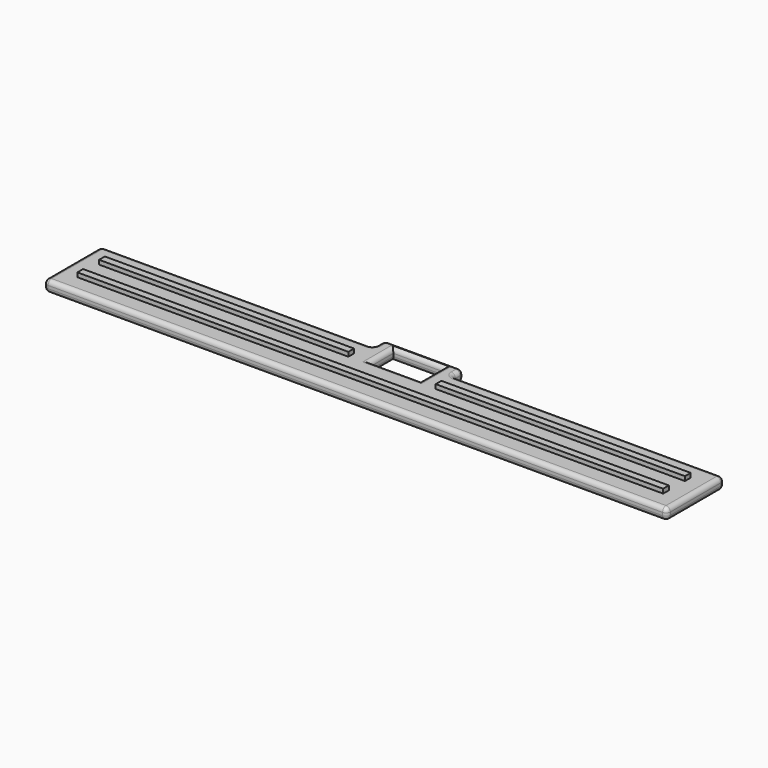
from build123d import *

# Parameters (mm, degrees)
F0_W          = 7
F0_H          = 4
F1_DEPTH      = 1.6
F2_T3_DEPTH   = 1.6
F2_T6_DEPTH   = 1.6
F2_S9_W       = 0.6
F2_S9_H       = 0.6
F2_T10_DEPTH  = 0.6
F2_S14_W      = 0.6
F2_S14_H      = 0.6
F2_T15_DEPTH  = 0.6
F2_S19_W      = 0.6
F2_S19_H      = 0.6
F2_T20_DEPTH  = 0.6
F2_S24_W      = 0.6
F2_S24_H      = 0.6
F2_T25_DEPTH  = 0.6
F2_T30_DEPTH  = 10.9
F2_T33_DEPTH  = 85.8
F2_T36_DEPTH  = 10.9
F2_T39_DEPTH  = 14
F2_T42_DEPTH  = 4
F2_T45_DEPTH  = 7
F2_T48_DEPTH  = 4
F2_T51_DEPTH  = 7
F2_T54_DEPTH  = 10.9
F2_T57_DEPTH  = 85.8
F2_T60_DEPTH  = 10.9
F2_T63_DEPTH  = 14
F2_T66_DEPTH  = 4
F2_T69_DEPTH  = 7
F2_T72_DEPTH  = 4
F2_T75_DEPTH  = 7
F2_T78_DEPTH  = 0.4
F2_T81_DEPTH  = 4.6
F2_T84_DEPTH  = 4.6
F2_T87_DEPTH  = 4.6
F2_T90_DEPTH  = 4.6
F2_T93_DEPTH  = 0.4
F2_T97_DEPTH  = 5.5
F2_T101_DEPTH = 8.5
F2_T107_DEPTH = 5.5
F2_T111_DEPTH = 8.5
F2_T117_DEPTH = 8.5
F2_T121_DEPTH = 5.5
F2_T127_DEPTH = 5.5
F2_T131_DEPTH = 8.5
F2_T137_DEPTH = 5.5
F2_T141_DEPTH = 8.5
F2_T147_DEPTH = 5.5
F2_T151_DEPTH = 8.5
F2_T157_DEPTH = 8.5
F2_T161_DEPTH = 5.5
F2_T167_DEPTH = 5.5
F2_T171_DEPTH = 8.5
F2_S176_W     = 0.6
F2_S176_H     = 0.6
F2_T177_DEPTH = 0.6
F2_S181_W     = 0.6
F2_S181_H     = 0.6
F2_T182_DEPTH = 0.6
F2_S186_W     = 0.6
F2_S186_H     = 0.6
F2_T187_DEPTH = 0.6
F2_S191_W     = 0.6
F2_S191_H     = 0.6
F2_T192_DEPTH = 0.6
F2_S196_W     = 0.6
F2_S196_H     = 0.6
F2_T197_DEPTH = 0.6
F2_S201_W     = 0.6
F2_S201_H     = 0.6
F2_T202_DEPTH = 0.6
F2_S206_W     = 0.6
F2_S206_H     = 0.6
F2_T207_DEPTH = 0.6
F2_S211_W     = 0.6
F2_S211_H     = 0.6
F2_T212_DEPTH = 0.6
F2_T217_DEPTH = 36.8
F2_T220_DEPTH = 0.8
F2_T223_DEPTH = 0.8
F2_T226_DEPTH = 36.8
F2_T229_DEPTH = 36.8
F2_T232_DEPTH = 0.8
F2_T235_DEPTH = 0.8
F2_T238_DEPTH = 36.8
F2_T241_ANGLE = 90
F2_T244_ANGLE = 90
F2_T247_ANGLE = 90
F2_T250_ANGLE = 90
F3_W          = 34.8
F3_H          = 1
F3_W_2        = 81.8
F4_DEPTH      = 2.2


# Not quite as in the source:
# - a fillet or chamfer that OpenCascade refuses, or shapes differently, is made with other operations: its cross-section is extruded or revolved along the edge and cut away or added


with BuildPart() as f1:
    # F0 (on Top) → F1 (new body)
    with BuildSketch(Plane.XY):
        Polygon((-43.5, 10), (-43.5, 0), (43.5, 0), (43.5, 10), (5.5, 10), (5.5, 12), (-5.5, 12), (-5.5, 10), align=None)
        with Locations((0, 9)):
            Rectangle(F0_W, F0_H, mode=Mode.SUBTRACT)
    extrude(amount=F1_DEPTH)

    # F2: fillet of radius 0.6 on 32 edges, made by hand


with BuildPart() as f2_tool1:
    # F2_s2 → F2_t3 (new body)
    with BuildSketch(Plane.XY):
        with BuildLine():
            ThreePointArc((6.1, 10), (5.6757359313, 10.1757359313), (5.5, 10.6))
            Line((5.5, 10.6), (5.5, 10))
            Line((5.5, 10), (6.1, 10))
        make_face()
    extrude(amount=F2_T3_DEPTH)


with BuildPart() as f2_tool4:
    # F2_s5 → F2_t6 (new body)
    with BuildSketch(Plane.XY):
        with BuildLine():
            ThreePointArc((-5.5, 10.6), (-5.6757359313, 10.1757359313), (-6.1, 10))
            Line((-6.1, 10), (-5.5, 10))
            Line((-5.5, 10), (-5.5, 10.6))
        make_face()
    extrude(amount=F2_T6_DEPTH)


with BuildPart() as f1_1:
    add(f1.part)

    # F2_t7: union F2_tool1, F2_tool4
    add([f2_tool1.part, f2_tool4.part])


with BuildPart() as f2_tool8:
    # F2_s9 → F2_t10 (new body)
    with BuildSketch(Plane.YZ.offset(-42.9)):
        with Locations((0.3, 1.3)):
            Rectangle(F2_S9_W, F2_S9_H)
    extrude(amount=-F2_T10_DEPTH)

    # F2_s11 → F2_t12 (revolve, cut)
    with BuildSketch(Plane(origin=(-42.9, 0.6, 1), x_dir=(0, 0.7071067812, -0.7071067812), z_dir=(0, 0.7071067812, 0.7071067812))):
        with BuildLine():
            ThreePointArc((0, -0.6), (0.6, 0), (0, 0.6))
            Line((0, 0.6), (0, -0.6))
        make_face()
    revolve(axis=Axis((-42.9, 0.6, 1), (-1, 0, 0)), mode=Mode.SUBTRACT)


with BuildPart() as f2_tool13:
    # F2_s14 → F2_t15 (new body)
    with BuildSketch(Plane.XZ.offset(-0.6)):
        with Locations((43.2, 1.3)):
            Rectangle(F2_S14_W, F2_S14_H)
    extrude(amount=F2_T15_DEPTH)

    # F2_s16 → F2_t17 (revolve, cut)
    with BuildSketch(Plane(origin=(42.9, 0.6, 1), x_dir=(-0.7071067812, 0, -0.7071067812), z_dir=(-0.7071067812, 0, 0.7071067812))):
        with BuildLine():
            ThreePointArc((0, -0.6), (0.6, 0), (0, 0.6))
            Line((0, 0.6), (0, -0.6))
        make_face()
    revolve(axis=Axis((42.9, 0.6, 1), (0, -1, 0)), mode=Mode.SUBTRACT)


with BuildPart() as f2_tool18:
    # F2_s19 → F2_t20 (new body)
    with BuildSketch(Plane.YZ.offset(-42.9)):
        with Locations((0.3, 0.3)):
            Rectangle(F2_S19_W, F2_S19_H)
    extrude(amount=-F2_T20_DEPTH)

    # F2_s21 → F2_t22 (revolve, cut)
    with BuildSketch(Plane(origin=(-42.9, 0.6, 0.6), x_dir=(0, 0.7071067812, 0.7071067812), z_dir=(0, -0.7071067812, 0.7071067812))):
        with BuildLine():
            ThreePointArc((0, -0.6), (0.6, 0), (0, 0.6))
            Line((0, 0.6), (0, -0.6))
        make_face()
    revolve(axis=Axis((-42.9, 0.6, 0.6), (-1, 0, 0)), mode=Mode.SUBTRACT)


with BuildPart() as f2_tool23:
    # F2_s24 → F2_t25 (new body)
    with BuildSketch(Plane.XZ.offset(-0.6)):
        with Locations((43.2, 0.3)):
            Rectangle(F2_S24_W, F2_S24_H)
    extrude(amount=F2_T25_DEPTH)

    # F2_s26 → F2_t27 (revolve, cut)
    with BuildSketch(Plane(origin=(42.9, 0.6, 0.6), x_dir=(-0.7071067812, 0, 0.7071067812), z_dir=(0.7071067812, 0, 0.7071067812))):
        with BuildLine():
            ThreePointArc((0, -0.6), (0.6, 0), (0, 0.6))
            Line((0, 0.6), (0, -0.6))
        make_face()
    revolve(axis=Axis((42.9, 0.6, 0.6), (0, -1, 0)), mode=Mode.SUBTRACT)


with BuildPart() as f2_tool28:
    # F2_s29 → F2_t30 (new body)
    with BuildSketch(Plane.XZ.offset(-11.5)):
        with BuildLine():
            ThreePointArc((-43.5, 1), (-43.3242640687, 1.4242640687), (-42.9, 1.6))
            Line((-42.9, 1.6), (-43.5, 1.6))
            Line((-43.5, 1.6), (-43.5, 1))
        make_face()
    extrude(amount=F2_T30_DEPTH)


with BuildPart() as f2_tool31:
    # F2_s32 → F2_t33 (new body)
    with BuildSketch(Plane.YZ.offset(-42.9)):
        with BuildLine():
            ThreePointArc((0, 1), (0.1757359313, 1.4242640687), (0.6, 1.6))
            Line((0.6, 1.6), (0, 1.6))
            Line((0, 1.6), (0, 1))
        make_face()
    extrude(amount=F2_T33_DEPTH)


with BuildPart() as f2_tool34:
    # F2_s35 → F2_t36 (new body)
    with BuildSketch(Plane.XZ.offset(-0.6)):
        with BuildLine():
            ThreePointArc((42.9, 1.6), (43.3242640687, 1.4242640687), (43.5, 1))
            Line((43.5, 1), (43.5, 1.6))
            Line((43.5, 1.6), (42.9, 1.6))
        make_face()
    extrude(amount=-F2_T36_DEPTH)


with BuildPart() as f2_tool37:
    # F2_s38 → F2_t39 (new body)
    with BuildSketch(Plane.YZ.offset(7)):
        with BuildLine():
            ThreePointArc((11.4, 1.6), (11.8242640687, 1.4242640687), (12, 1))
            Line((12, 1), (12, 1.6))
            Line((12, 1.6), (11.4, 1.6))
        make_face()
    extrude(amount=-F2_T39_DEPTH)


with BuildPart() as f2_tool40:
    # F2_s41 → F2_t42 (new body)
    with BuildSketch(Plane.XZ.offset(-7)):
        with BuildLine():
            ThreePointArc((-4.1, 1.6), (-3.6757359313, 1.4242640687), (-3.5, 1))
            Line((-3.5, 1), (-3.5, 1.6))
            Line((-3.5, 1.6), (-4.1, 1.6))
        make_face()
    extrude(amount=-F2_T42_DEPTH)


with BuildPart() as f2_tool43:
    # F2_s44 → F2_t45 (new body)
    with BuildSketch(Plane.YZ.offset(-3.5)):
        with BuildLine():
            ThreePointArc((11.6, 1.6), (11.1757359313, 1.4242640687), (11, 1))
            Line((11, 1), (11, 1.6))
            Line((11, 1.6), (11.6, 1.6))
        make_face()
    extrude(amount=F2_T45_DEPTH)


with BuildPart() as f2_tool46:
    # F2_s47 → F2_t48 (new body)
    with BuildSketch(Plane.XZ.offset(-11)):
        with BuildLine():
            ThreePointArc((4.1, 1.6), (3.6757359313, 1.4242640687), (3.5, 1))
            Line((3.5, 1), (3.5, 1.6))
            Line((3.5, 1.6), (4.1, 1.6))
        make_face()
    extrude(amount=F2_T48_DEPTH)


with BuildPart() as f2_tool49:
    # F2_s50 → F2_t51 (new body)
    with BuildSketch(Plane.YZ.offset(3.5)):
        with BuildLine():
            ThreePointArc((6.4, 1.6), (6.8242640687, 1.4242640687), (7, 1))
            Line((7, 1), (7, 1.6))
            Line((7, 1.6), (6.4, 1.6))
        make_face()
    extrude(amount=-F2_T51_DEPTH)


with BuildPart() as f2_tool52:
    # F2_s53 → F2_t54 (new body)
    with BuildSketch(Plane.XZ.offset(-11.5)):
        with BuildLine():
            ThreePointArc((-43.5, 0.6), (-43.3242640687, 0.1757359313), (-42.9, 0))
            Line((-42.9, 0), (-43.5, 0))
            Line((-43.5, 0), (-43.5, 0.6))
        make_face()
    extrude(amount=F2_T54_DEPTH)


with BuildPart() as f2_tool55:
    # F2_s56 → F2_t57 (new body)
    with BuildSketch(Plane.YZ.offset(-42.9)):
        with BuildLine():
            ThreePointArc((0, 0.6), (0.1757359313, 0.1757359313), (0.6, 0))
            Line((0.6, 0), (0, 0))
            Line((0, 0), (0, 0.6))
        make_face()
    extrude(amount=F2_T57_DEPTH)


with BuildPart() as f2_tool58:
    # F2_s59 → F2_t60 (new body)
    with BuildSketch(Plane.XZ.offset(-0.6)):
        with BuildLine():
            ThreePointArc((42.9, 0), (43.3242640687, 0.1757359313), (43.5, 0.6))
            Line((43.5, 0.6), (43.5, 0))
            Line((43.5, 0), (42.9, 0))
        make_face()
    extrude(amount=-F2_T60_DEPTH)


with BuildPart() as f2_tool61:
    # F2_s62 → F2_t63 (new body)
    with BuildSketch(Plane.YZ.offset(7)):
        with BuildLine():
            ThreePointArc((11.4, 0), (11.8242640687, 0.1757359313), (12, 0.6))
            Line((12, 0.6), (12, 0))
            Line((12, 0), (11.4, 0))
        make_face()
    extrude(amount=-F2_T63_DEPTH)


with BuildPart() as f2_tool64:
    # F2_s65 → F2_t66 (new body)
    with BuildSketch(Plane.XZ.offset(-7)):
        with BuildLine():
            ThreePointArc((-4.1, 0), (-3.6757359313, 0.1757359313), (-3.5, 0.6))
            Line((-3.5, 0.6), (-3.5, 0))
            Line((-3.5, 0), (-4.1, 0))
        make_face()
    extrude(amount=-F2_T66_DEPTH)


with BuildPart() as f2_tool67:
    # F2_s68 → F2_t69 (new body)
    with BuildSketch(Plane.YZ.offset(-3.5)):
        with BuildLine():
            ThreePointArc((11.6, 0), (11.1757359313, 0.1757359313), (11, 0.6))
            Line((11, 0.6), (11, 0))
            Line((11, 0), (11.6, 0))
        make_face()
    extrude(amount=F2_T69_DEPTH)


with BuildPart() as f2_tool70:
    # F2_s71 → F2_t72 (new body)
    with BuildSketch(Plane.XZ.offset(-11)):
        with BuildLine():
            ThreePointArc((4.1, 0), (3.6757359313, 0.1757359313), (3.5, 0.6))
            Line((3.5, 0.6), (3.5, 0))
            Line((3.5, 0), (4.1, 0))
        make_face()
    extrude(amount=F2_T72_DEPTH)


with BuildPart() as f2_tool73:
    # F2_s74 → F2_t75 (new body)
    with BuildSketch(Plane.YZ.offset(3.5)):
        with BuildLine():
            ThreePointArc((6.4, 0), (6.8242640687, 0.1757359313), (7, 0.6))
            Line((7, 0.6), (7, 0))
            Line((7, 0), (6.4, 0))
        make_face()
    extrude(amount=-F2_T75_DEPTH)


with BuildPart() as f2_tool76:
    # F2_s77 → F2_t78 (new body)
    with BuildSketch(Plane.XY.offset(0.6)):
        with BuildLine():
            ThreePointArc((42.9, 0), (43.3242640687, 0.1757359313), (43.5, 0.6))
            Line((43.5, 0.6), (43.5, 0))
            Line((43.5, 0), (42.9, 0))
        make_face()
    extrude(amount=F2_T78_DEPTH)


with BuildPart() as f2_tool79:
    # F2_s80 → F2_t81 (new body)
    with BuildSketch(Plane.XY.offset(-1.5)):
        with BuildLine():
            ThreePointArc((43.5, 9.4), (43.3242640687, 9.8242640687), (42.9, 10))
            Line((42.9, 10), (43.5, 10))
            Line((43.5, 10), (43.5, 9.4))
        make_face()
    extrude(amount=F2_T81_DEPTH)


with BuildPart() as f2_tool82:
    # F2_s83 → F2_t84 (new body)
    with BuildSketch(Plane.XY.offset(-1.5)):
        with BuildLine():
            ThreePointArc((5.5, 11.4), (5.3242640687, 11.8242640687), (4.9, 12))
            Line((4.9, 12), (5.5, 12))
            Line((5.5, 12), (5.5, 11.4))
        make_face()
    extrude(amount=F2_T84_DEPTH)


with BuildPart() as f2_tool85:
    # F2_s86 → F2_t87 (new body)
    with BuildSketch(Plane.XY.offset(-1.5)):
        with BuildLine():
            ThreePointArc((-4.9, 12), (-5.3242640687, 11.8242640687), (-5.5, 11.4))
            Line((-5.5, 11.4), (-5.5, 12))
            Line((-5.5, 12), (-4.9, 12))
        make_face()
    extrude(amount=F2_T87_DEPTH)


with BuildPart() as f2_tool88:
    # F2_s89 → F2_t90 (new body)
    with BuildSketch(Plane.XY.offset(-1.5)):
        with BuildLine():
            ThreePointArc((-43.5, 9.4), (-43.3242640687, 9.8242640687), (-42.9, 10))
            Line((-42.9, 10), (-43.5, 10))
            Line((-43.5, 10), (-43.5, 9.4))
        make_face()
    extrude(amount=F2_T90_DEPTH)


with BuildPart() as f2_tool91:
    # F2_s92 → F2_t93 (new body)
    with BuildSketch(Plane.XY.offset(0.6)):
        with BuildLine():
            ThreePointArc((-43.5, 0.6), (-43.3242640687, 0.1757359313), (-42.9, 0))
            Line((-42.9, 0), (-43.5, 0))
            Line((-43.5, 0), (-43.5, 0.6))
        make_face()
    extrude(amount=F2_T93_DEPTH)


with BuildPart() as f2_tool95:
    # F2_s96 → F2_t97 (new body)
    with BuildSketch(Plane.XZ.offset(-5.5)):
        with BuildLine():
            ThreePointArc((-4.1, 1.6), (-3.6757359313, 1.4242640687), (-3.5, 1))
            Line((-3.5, 1), (-3.5, 1.6))
            Line((-3.5, 1.6), (-4.1, 1.6))
        make_face()
    extrude(amount=-F2_T97_DEPTH)

    split(bisect_by=Plane.XZ.offset(-7), keep=Keep.TOP)


with BuildPart() as f2_tool99:
    # F2_s100 → F2_t101 (new body)
    with BuildSketch(Plane.YZ.offset(3.5)):
        with BuildLine():
            ThreePointArc((6.4, 1.6), (6.8242640687, 1.4242640687), (7, 1))
            Line((7, 1), (7, 1.6))
            Line((7, 1.6), (6.4, 1.6))
        make_face()
    extrude(amount=-F2_T101_DEPTH)

    split(bisect_by=Plane.YZ.offset(-3.5), keep=Keep.BOTTOM)


with BuildPart() as f2_tool95_1:
    add(f2_tool95.part)

    # F2_t103: intersect F2_tool99
    add(f2_tool99.part, mode=Mode.INTERSECT)


with BuildPart() as f2_tool105:
    # F2_s106 → F2_t107 (new body)
    with BuildSketch(Plane.XZ.offset(-7)):
        with BuildLine():
            ThreePointArc((-4.1, 1.6), (-3.6757359313, 1.4242640687), (-3.5, 1))
            Line((-3.5, 1), (-3.5, 1.6))
            Line((-3.5, 1.6), (-4.1, 1.6))
        make_face()
    extrude(amount=-F2_T107_DEPTH)

    split(bisect_by=Plane.XZ.offset(-11), keep=Keep.BOTTOM)


with BuildPart() as f2_tool109:
    # F2_s110 → F2_t111 (new body)
    with BuildSketch(Plane.YZ.offset(-5)):
        with BuildLine():
            ThreePointArc((11.6, 1.6), (11.1757359313, 1.4242640687), (11, 1))
            Line((11, 1), (11, 1.6))
            Line((11, 1.6), (11.6, 1.6))
        make_face()
    extrude(amount=F2_T111_DEPTH)

    split(bisect_by=Plane.YZ.offset(-3.5), keep=Keep.BOTTOM)


with BuildPart() as f2_tool105_1:
    add(f2_tool105.part)

    # F2_t113: intersect F2_tool109
    add(f2_tool109.part, mode=Mode.INTERSECT)


with BuildPart() as f2_tool115:
    # F2_s116 → F2_t117 (new body)
    with BuildSketch(Plane.YZ.offset(-3.5)):
        with BuildLine():
            ThreePointArc((11.6, 1.6), (11.1757359313, 1.4242640687), (11, 1))
            Line((11, 1), (11, 1.6))
            Line((11, 1.6), (11.6, 1.6))
        make_face()
    extrude(amount=F2_T117_DEPTH)

    split(bisect_by=Plane.YZ.offset(3.5), keep=Keep.TOP)


with BuildPart() as f2_tool119:
    # F2_s120 → F2_t121 (new body)
    with BuildSketch(Plane.XZ.offset(-12.5)):
        with BuildLine():
            ThreePointArc((4.1, 1.6), (3.6757359313, 1.4242640687), (3.5, 1))
            Line((3.5, 1), (3.5, 1.6))
            Line((3.5, 1.6), (4.1, 1.6))
        make_face()
    extrude(amount=F2_T121_DEPTH)

    split(bisect_by=Plane.XZ.offset(-11), keep=Keep.BOTTOM)


with BuildPart() as f2_tool115_1:
    add(f2_tool115.part)

    # F2_t123: intersect F2_tool119
    add(f2_tool119.part, mode=Mode.INTERSECT)


with BuildPart() as f2_tool125:
    # F2_s126 → F2_t127 (new body)
    with BuildSketch(Plane.XZ.offset(-11)):
        with BuildLine():
            ThreePointArc((4.1, 1.6), (3.6757359313, 1.4242640687), (3.5, 1))
            Line((3.5, 1), (3.5, 1.6))
            Line((3.5, 1.6), (4.1, 1.6))
        make_face()
    extrude(amount=F2_T127_DEPTH)

    split(bisect_by=Plane.XZ.offset(-7), keep=Keep.TOP)


with BuildPart() as f2_tool129:
    # F2_s130 → F2_t131 (new body)
    with BuildSketch(Plane.YZ.offset(5)):
        with BuildLine():
            ThreePointArc((6.4, 1.6), (6.8242640687, 1.4242640687), (7, 1))
            Line((7, 1), (7, 1.6))
            Line((7, 1.6), (6.4, 1.6))
        make_face()
    extrude(amount=-F2_T131_DEPTH)

    split(bisect_by=Plane.YZ.offset(3.5), keep=Keep.TOP)


with BuildPart() as f2_tool125_1:
    add(f2_tool125.part)

    # F2_t133: intersect F2_tool129
    add(f2_tool129.part, mode=Mode.INTERSECT)


with BuildPart() as f2_tool135:
    # F2_s136 → F2_t137 (new body)
    with BuildSketch(Plane.XZ.offset(-5.5)):
        with BuildLine():
            ThreePointArc((-4.1, 0), (-3.6757359313, 0.1757359313), (-3.5, 0.6))
            Line((-3.5, 0.6), (-3.5, 0))
            Line((-3.5, 0), (-4.1, 0))
        make_face()
    extrude(amount=-F2_T137_DEPTH)

    split(bisect_by=Plane.XZ.offset(-7), keep=Keep.TOP)


with BuildPart() as f2_tool139:
    # F2_s140 → F2_t141 (new body)
    with BuildSketch(Plane.YZ.offset(3.5)):
        with BuildLine():
            ThreePointArc((6.4, 0), (6.8242640687, 0.1757359313), (7, 0.6))
            Line((7, 0.6), (7, 0))
            Line((7, 0), (6.4, 0))
        make_face()
    extrude(amount=-F2_T141_DEPTH)

    split(bisect_by=Plane.YZ.offset(-3.5), keep=Keep.BOTTOM)


with BuildPart() as f2_tool135_1:
    add(f2_tool135.part)

    # F2_t143: intersect F2_tool139
    add(f2_tool139.part, mode=Mode.INTERSECT)


with BuildPart() as f2_tool145:
    # F2_s146 → F2_t147 (new body)
    with BuildSketch(Plane.XZ.offset(-7)):
        with BuildLine():
            ThreePointArc((-4.1, 0), (-3.6757359313, 0.1757359313), (-3.5, 0.6))
            Line((-3.5, 0.6), (-3.5, 0))
            Line((-3.5, 0), (-4.1, 0))
        make_face()
    extrude(amount=-F2_T147_DEPTH)

    split(bisect_by=Plane.XZ.offset(-11), keep=Keep.BOTTOM)


with BuildPart() as f2_tool149:
    # F2_s150 → F2_t151 (new body)
    with BuildSketch(Plane.YZ.offset(-5)):
        with BuildLine():
            ThreePointArc((11.6, 0), (11.1757359313, 0.1757359313), (11, 0.6))
            Line((11, 0.6), (11, 0))
            Line((11, 0), (11.6, 0))
        make_face()
    extrude(amount=F2_T151_DEPTH)

    split(bisect_by=Plane.YZ.offset(-3.5), keep=Keep.BOTTOM)


with BuildPart() as f2_tool145_1:
    add(f2_tool145.part)

    # F2_t153: intersect F2_tool149
    add(f2_tool149.part, mode=Mode.INTERSECT)


with BuildPart() as f2_tool155:
    # F2_s156 → F2_t157 (new body)
    with BuildSketch(Plane.YZ.offset(-3.5)):
        with BuildLine():
            ThreePointArc((11.6, 0), (11.1757359313, 0.1757359313), (11, 0.6))
            Line((11, 0.6), (11, 0))
            Line((11, 0), (11.6, 0))
        make_face()
    extrude(amount=F2_T157_DEPTH)

    split(bisect_by=Plane.YZ.offset(3.5), keep=Keep.TOP)


with BuildPart() as f2_tool159:
    # F2_s160 → F2_t161 (new body)
    with BuildSketch(Plane.XZ.offset(-12.5)):
        with BuildLine():
            ThreePointArc((4.1, 0), (3.6757359313, 0.1757359313), (3.5, 0.6))
            Line((3.5, 0.6), (3.5, 0))
            Line((3.5, 0), (4.1, 0))
        make_face()
    extrude(amount=F2_T161_DEPTH)

    split(bisect_by=Plane.XZ.offset(-11), keep=Keep.BOTTOM)


with BuildPart() as f2_tool155_1:
    add(f2_tool155.part)

    # F2_t163: intersect F2_tool159
    add(f2_tool159.part, mode=Mode.INTERSECT)


with BuildPart() as f2_tool165:
    # F2_s166 → F2_t167 (new body)
    with BuildSketch(Plane.XZ.offset(-11)):
        with BuildLine():
            ThreePointArc((4.1, 0), (3.6757359313, 0.1757359313), (3.5, 0.6))
            Line((3.5, 0.6), (3.5, 0))
            Line((3.5, 0), (4.1, 0))
        make_face()
    extrude(amount=F2_T167_DEPTH)

    split(bisect_by=Plane.XZ.offset(-7), keep=Keep.TOP)


with BuildPart() as f2_tool169:
    # F2_s170 → F2_t171 (new body)
    with BuildSketch(Plane.YZ.offset(5)):
        with BuildLine():
            ThreePointArc((6.4, 0), (6.8242640687, 0.1757359313), (7, 0.6))
            Line((7, 0.6), (7, 0))
            Line((7, 0), (6.4, 0))
        make_face()
    extrude(amount=-F2_T171_DEPTH)

    split(bisect_by=Plane.YZ.offset(3.5), keep=Keep.TOP)


with BuildPart() as f2_tool165_1:
    add(f2_tool165.part)

    # F2_t173: intersect F2_tool169
    add(f2_tool169.part, mode=Mode.INTERSECT)


with BuildPart() as f1_2:
    add(f1_1.part)

    # F2_t174: cut F2_tool8, F2_tool13, F2_tool18, F2_tool23, F2_tool28, F2_tool31, F2_tool34, F2_tool37, F2_tool40, F2_tool43, F2_tool46, F2_tool49, F2_tool52, F2_tool55, F2_tool58, F2_tool61, F2_tool64, F2_tool67, F2_tool70, F2_tool73, F2_tool76, F2_tool79, F2_tool82, F2_tool85, F2_tool88, F2_tool91, F2_tool95, F2_tool105, F2_tool115, F2_tool125, F2_tool135, F2_tool145, F2_tool155, F2_tool165
    add([f2_tool8.part, f2_tool13.part, f2_tool18.part, f2_tool23.part, f2_tool28.part, f2_tool31.part, f2_tool34.part, f2_tool37.part, f2_tool40.part, f2_tool43.part, f2_tool46.part, f2_tool49.part, f2_tool52.part, f2_tool55.part, f2_tool58.part, f2_tool61.part, f2_tool64.part, f2_tool67.part, f2_tool70.part, f2_tool73.part, f2_tool76.part, f2_tool79.part, f2_tool82.part, f2_tool85.part, f2_tool88.part, f2_tool91.part, f2_tool95_1.part, f2_tool105_1.part, f2_tool115_1.part, f2_tool125_1.part, f2_tool135_1.part, f2_tool145_1.part, f2_tool155_1.part, f2_tool165_1.part], mode=Mode.SUBTRACT)


with BuildPart() as f2_tool175:
    # F2_s176 → F2_t177 (new body)
    with BuildSketch(Plane.XZ.offset(-9.4)):
        with Locations((-43.2, 0.3)):
            Rectangle(F2_S176_W, F2_S176_H)
    extrude(amount=-F2_T177_DEPTH)

    # F2_s178 → F2_t179 (revolve, cut)
    with BuildSketch(Plane(origin=(-42.9, 9.4, 0.6), x_dir=(0.7071067812, 0, 0.7071067812), z_dir=(-0.7071067812, 0, 0.7071067812))):
        with BuildLine():
            ThreePointArc((0, -0.6), (0.6, 0), (0, 0.6))
            Line((0, 0.6), (0, -0.6))
        make_face()
    revolve(axis=Axis((-42.9, 9.4, 0.6), (0, 1, 0)), mode=Mode.SUBTRACT)


with BuildPart() as f2_tool180:
    # F2_s181 → F2_t182 (new body)
    with BuildSketch(Plane.YZ.offset(-4.9)):
        with Locations((11.7, 0.3)):
            Rectangle(F2_S181_W, F2_S181_H)
    extrude(amount=-F2_T182_DEPTH)

    # F2_s183 → F2_t184 (revolve, cut)
    with BuildSketch(Plane(origin=(-4.9, 11.4, 0.6), x_dir=(0, -0.7071067812, 0.7071067812), z_dir=(0, -0.7071067812, -0.7071067812))):
        with BuildLine():
            ThreePointArc((0, -0.6), (0.6, 0), (0, 0.6))
            Line((0, 0.6), (0, -0.6))
        make_face()
    revolve(axis=Axis((-4.9, 11.4, 0.6), (-1, 0, 0)), mode=Mode.SUBTRACT)


with BuildPart() as f2_tool185:
    # F2_s186 → F2_t187 (new body)
    with BuildSketch(Plane.YZ.offset(4.9)):
        with Locations((11.7, 0.3)):
            Rectangle(F2_S186_W, F2_S186_H)
    extrude(amount=F2_T187_DEPTH)

    # F2_s188 → F2_t189 (revolve, cut)
    with BuildSketch(Plane(origin=(4.9, 11.4, 0.6), x_dir=(0, -0.7071067812, 0.7071067812), z_dir=(0, 0.7071067812, 0.7071067812))):
        with BuildLine():
            ThreePointArc((0, -0.6), (0.6, 0), (0, 0.6))
            Line((0, 0.6), (0, -0.6))
        make_face()
    revolve(axis=Axis((4.9, 11.4, 0.6), (1, 0, 0)), mode=Mode.SUBTRACT)


with BuildPart() as f2_tool190:
    # F2_s191 → F2_t192 (new body)
    with BuildSketch(Plane.XZ.offset(-9.4)):
        with Locations((43.2, 0.3)):
            Rectangle(F2_S191_W, F2_S191_H)
    extrude(amount=-F2_T192_DEPTH)

    # F2_s193 → F2_t194 (revolve, cut)
    with BuildSketch(Plane(origin=(42.9, 9.4, 0.6), x_dir=(-0.7071067812, 0, 0.7071067812), z_dir=(-0.7071067812, 0, -0.7071067812))):
        with BuildLine():
            ThreePointArc((0, -0.6), (0.6, 0), (0, 0.6))
            Line((0, 0.6), (0, -0.6))
        make_face()
    revolve(axis=Axis((42.9, 9.4, 0.6), (0, 1, 0)), mode=Mode.SUBTRACT)


with BuildPart() as f2_tool195:
    # F2_s196 → F2_t197 (new body)
    with BuildSketch(Plane.XZ.offset(-9.4)):
        with Locations((-43.2, 1.3)):
            Rectangle(F2_S196_W, F2_S196_H)
    extrude(amount=-F2_T197_DEPTH)

    # F2_s198 → F2_t199 (revolve, cut)
    with BuildSketch(Plane(origin=(-42.9, 9.4, 1), x_dir=(0.7071067812, 0, -0.7071067812), z_dir=(0.7071067812, 0, 0.7071067812))):
        with BuildLine():
            ThreePointArc((0, -0.6), (0.6, 0), (0, 0.6))
            Line((0, 0.6), (0, -0.6))
        make_face()
    revolve(axis=Axis((-42.9, 9.4, 1), (0, 1, 0)), mode=Mode.SUBTRACT)


with BuildPart() as f2_tool200:
    # F2_s201 → F2_t202 (new body)
    with BuildSketch(Plane.YZ.offset(-4.9)):
        with Locations((11.7, 1.3)):
            Rectangle(F2_S201_W, F2_S201_H)
    extrude(amount=-F2_T202_DEPTH)

    # F2_s203 → F2_t204 (revolve, cut)
    with BuildSketch(Plane(origin=(-4.9, 11.4, 1), x_dir=(0, -0.7071067812, -0.7071067812), z_dir=(0, 0.7071067812, -0.7071067812))):
        with BuildLine():
            ThreePointArc((0, -0.6), (0.6, 0), (0, 0.6))
            Line((0, 0.6), (0, -0.6))
        make_face()
    revolve(axis=Axis((-4.9, 11.4, 1), (-1, 0, 0)), mode=Mode.SUBTRACT)


with BuildPart() as f2_tool205:
    # F2_s206 → F2_t207 (new body)
    with BuildSketch(Plane.YZ.offset(4.9)):
        with Locations((11.7, 1.3)):
            Rectangle(F2_S206_W, F2_S206_H)
    extrude(amount=F2_T207_DEPTH)

    # F2_s208 → F2_t209 (revolve, cut)
    with BuildSketch(Plane(origin=(4.9, 11.4, 1), x_dir=(0, -0.7071067812, -0.7071067812), z_dir=(0, -0.7071067812, 0.7071067812))):
        with BuildLine():
            ThreePointArc((0, -0.6), (0.6, 0), (0, 0.6))
            Line((0, 0.6), (0, -0.6))
        make_face()
    revolve(axis=Axis((4.9, 11.4, 1), (1, 0, 0)), mode=Mode.SUBTRACT)


with BuildPart() as f2_tool210:
    # F2_s211 → F2_t212 (new body)
    with BuildSketch(Plane.XZ.offset(-9.4)):
        with Locations((43.2, 1.3)):
            Rectangle(F2_S211_W, F2_S211_H)
    extrude(amount=-F2_T212_DEPTH)

    # F2_s213 → F2_t214 (revolve, cut)
    with BuildSketch(Plane(origin=(42.9, 9.4, 1), x_dir=(-0.7071067812, 0, -0.7071067812), z_dir=(0.7071067812, 0, -0.7071067812))):
        with BuildLine():
            ThreePointArc((0, -0.6), (0.6, 0), (0, 0.6))
            Line((0, 0.6), (0, -0.6))
        make_face()
    revolve(axis=Axis((42.9, 9.4, 1), (0, 1, 0)), mode=Mode.SUBTRACT)


with BuildPart() as f2_tool215:
    # F2_s216 → F2_t217 (new body)
    with BuildSketch(Plane.YZ.offset(42.9)):
        with BuildLine():
            ThreePointArc((10, 1), (9.8242640687, 1.4242640687), (9.4, 1.6))
            Line((9.4, 1.6), (10, 1.6))
            Line((10, 1.6), (10, 1))
        make_face()
    extrude(amount=-F2_T217_DEPTH)


with BuildPart() as f2_tool218:
    # F2_s219 → F2_t220 (new body)
    with BuildSketch(Plane.XZ.offset(-10.6)):
        with BuildLine():
            ThreePointArc((5.5, 1), (5.3242640687, 1.4242640687), (4.9, 1.6))
            Line((4.9, 1.6), (5.5, 1.6))
            Line((5.5, 1.6), (5.5, 1))
        make_face()
    extrude(amount=-F2_T220_DEPTH)


with BuildPart() as f2_tool221:
    # F2_s222 → F2_t223 (new body)
    with BuildSketch(Plane.XZ.offset(-11.4)):
        with BuildLine():
            ThreePointArc((-5.5, 1), (-5.3242640687, 1.4242640687), (-4.9, 1.6))
            Line((-4.9, 1.6), (-5.5, 1.6))
            Line((-5.5, 1.6), (-5.5, 1))
        make_face()
    extrude(amount=F2_T223_DEPTH)


with BuildPart() as f2_tool224:
    # F2_s225 → F2_t226 (new body)
    with BuildSketch(Plane.YZ.offset(-6.1)):
        with BuildLine():
            ThreePointArc((10, 1), (9.8242640687, 1.4242640687), (9.4, 1.6))
            Line((9.4, 1.6), (10, 1.6))
            Line((10, 1.6), (10, 1))
        make_face()
    extrude(amount=-F2_T226_DEPTH)


with BuildPart() as f2_tool227:
    # F2_s228 → F2_t229 (new body)
    with BuildSketch(Plane.YZ.offset(42.9)):
        with BuildLine():
            ThreePointArc((10, 0.6), (9.8242640687, 0.1757359313), (9.4, 0))
            Line((9.4, 0), (10, 0))
            Line((10, 0), (10, 0.6))
        make_face()
    extrude(amount=-F2_T229_DEPTH)


with BuildPart() as f2_tool230:
    # F2_s231 → F2_t232 (new body)
    with BuildSketch(Plane.XZ.offset(-10.6)):
        with BuildLine():
            ThreePointArc((5.5, 0.6), (5.3242640687, 0.1757359313), (4.9, 0))
            Line((4.9, 0), (5.5, 0))
            Line((5.5, 0), (5.5, 0.6))
        make_face()
    extrude(amount=-F2_T232_DEPTH)


with BuildPart() as f2_tool233:
    # F2_s234 → F2_t235 (new body)
    with BuildSketch(Plane.XZ.offset(-11.4)):
        with BuildLine():
            ThreePointArc((-5.5, 0.6), (-5.3242640687, 0.1757359313), (-4.9, 0))
            Line((-4.9, 0), (-5.5, 0))
            Line((-5.5, 0), (-5.5, 0.6))
        make_face()
    extrude(amount=F2_T235_DEPTH)


with BuildPart() as f2_tool236:
    # F2_s237 → F2_t238 (new body)
    with BuildSketch(Plane.YZ.offset(-6.1)):
        with BuildLine():
            ThreePointArc((10, 0.6), (9.8242640687, 0.1757359313), (9.4, 0))
            Line((9.4, 0), (10, 0))
            Line((10, 0), (10, 0.6))
        make_face()
    extrude(amount=-F2_T238_DEPTH)


with BuildPart() as f2_tool239:
    # F2_s240 → F2_t241 (revolve)
    with BuildSketch(Plane.XZ.offset(-10.6)):
        with BuildLine():
            ThreePointArc((-5.5, 0.6), (-5.3242640687, 0.1757359313), (-4.9, 0))
            Line((-4.9, 0), (-5.5, 0))
            Line((-5.5, 0), (-5.5, 0.6))
        make_face()
    revolve(axis=Axis((-6.1, 10.6, 0), (0, 0, -1)), revolution_arc=F2_T241_ANGLE)


with BuildPart() as f2_tool242:
    # F2_s243 → F2_t244 (revolve)
    with BuildSketch(Plane.YZ.offset(6.1)):
        with BuildLine():
            ThreePointArc((10, 0.6), (9.8242640687, 0.1757359313), (9.4, 0))
            Line((9.4, 0), (10, 0))
            Line((10, 0), (10, 0.6))
        make_face()
    revolve(axis=Axis((6.1, 10.6, 0), (0, 0, -1)), revolution_arc=F2_T244_ANGLE)


with BuildPart() as f2_tool245:
    # F2_s246 → F2_t247 (revolve)
    with BuildSketch(Plane.XZ.offset(-10.6)):
        with BuildLine():
            ThreePointArc((-5.5, 1), (-5.3242640687, 1.4242640687), (-4.9, 1.6))
            Line((-4.9, 1.6), (-5.5, 1.6))
            Line((-5.5, 1.6), (-5.5, 1))
        make_face()
    revolve(axis=Axis((-6.1, 10.6, 1.6), (0, 0, -1)), revolution_arc=F2_T247_ANGLE)


with BuildPart() as f2_tool248:
    # F2_s249 → F2_t250 (revolve)
    with BuildSketch(Plane.YZ.offset(6.1)):
        with BuildLine():
            ThreePointArc((10, 1), (9.8242640687, 1.4242640687), (9.4, 1.6))
            Line((9.4, 1.6), (10, 1.6))
            Line((10, 1.6), (10, 1))
        make_face()
    revolve(axis=Axis((6.1, 10.6, 1.6), (0, 0, -1)), revolution_arc=F2_T250_ANGLE)


with BuildPart() as f1_3:
    add(f1_2.part)

    # F2_t251: cut F2_tool175, F2_tool180, F2_tool185, F2_tool190, F2_tool195, F2_tool200, F2_tool205, F2_tool210, F2_tool215, F2_tool218, F2_tool221, F2_tool224, F2_tool227, F2_tool230, F2_tool233, F2_tool236, F2_tool239, F2_tool242, F2_tool245, F2_tool248
    add([f2_tool175.part, f2_tool180.part, f2_tool185.part, f2_tool190.part, f2_tool195.part, f2_tool200.part, f2_tool205.part, f2_tool210.part, f2_tool215.part, f2_tool218.part, f2_tool221.part, f2_tool224.part, f2_tool227.part, f2_tool230.part, f2_tool233.part, f2_tool236.part, f2_tool239.part, f2_tool242.part, f2_tool245.part, f2_tool248.part], mode=Mode.SUBTRACT)

    # F3 (on Top) → F4 (join)
    with BuildSketch(Plane.XY):
        with Locations((23.5, 6.9)):
            Rectangle(F3_W, F3_H)
        with Locations((0, 3.1)):
            Rectangle(F3_W_2, F3_H)
        with Locations((-23.5, 6.9)):
            Rectangle(F3_W, F3_H)
    extrude(amount=F4_DEPTH)


solid = f1_3.part
